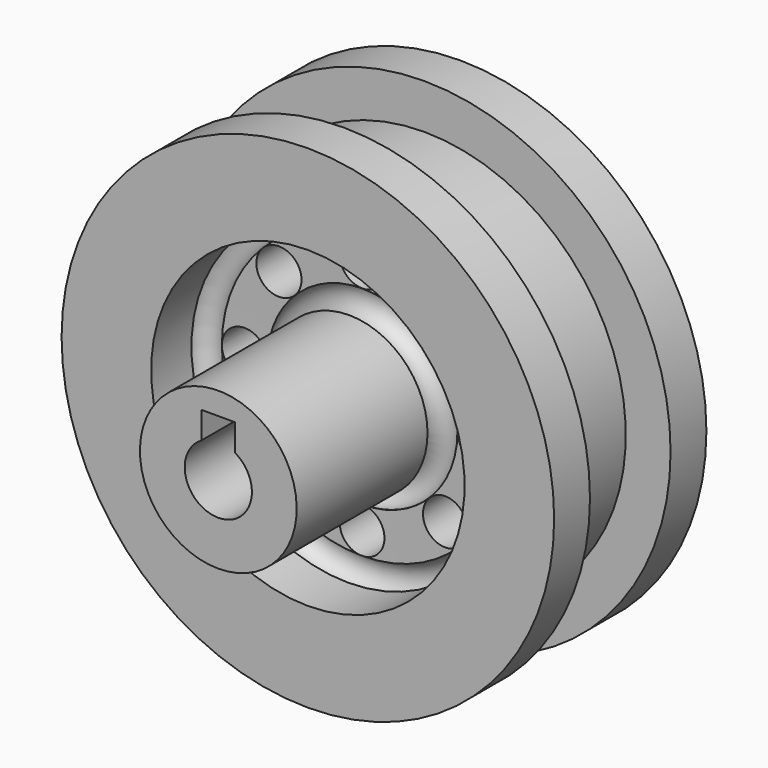
from build123d import *

# Parameters (mm, degrees)
F3_DEPTH        = 27.001
F4_R            = 2
F5_DEPTH        = 20.001
F5_COPIES_COUNT = 8
F6_R            = 1.5
F6_R_2          = 1.495


# Not quite as in the source:
# - a pattern or mirror of a feature is missing from the dataset's text; its kind, count and spacing are read off the source's solid


with BuildPart() as f1:
    # F0 (on Right) → F1 (revolve)
    with BuildSketch(Plane.YZ):
        Polygon((-11.6093918758, -7), (4.4935383189, -7), (4.3906081242, -13.9992432002), (-1.6093918758, -13.9992432002), (-1.6093918758, -21.9992432002), (2.3906081242, -21.9992432002), (2.3906081242, -17.9992432002), (11.3906081242, -17.9992432002), (11.3906081242, -21.9992432002), (15.3906081242, -21.9992432002), (15.3906081242, -13.9992432002), (8.3906081242, -13.9992432002), (8.3906081242, -7), (11.3906081242, -7), (11.3906081242, -3), (-11.6093918758, -3), align=None)
    revolve(axis=Axis((0, -0.5103430335, 0), (0, 1, 0)))

    # F2 (on face) → F3 (cut, through all)
    with BuildSketch(Plane.XZ.offset(11.6093918758)):
        with BuildLine():
            Line((-1.5, 5), (-1.5, 2.5980762114))
            ThreePointArc((-1.5, 2.5980762114), (0, 3), (1.5, 2.5980762114))
            Line((1.5, 2.5980762114), (1.5, 5))
            Line((1.5, 5), (-1.5, 5))
        make_face()
        with BuildLine():
            Line((-1.5, 2.5980762114), (-1.5, 0))
            Line((-1.5, 0), (1.5, 0))
            Line((1.5, 0), (1.5, 2.5980762114))
            ThreePointArc((1.5, 2.5980762114), (0, 3), (-1.5, 2.5980762114))
        make_face()
    extrude(amount=-F3_DEPTH, mode=Mode.SUBTRACT)

    # F4 (on face) → F5 (cut, through all)
    with BuildSketch(Plane(origin=(0, 8.3906081242, 0), x_dir=(-1, 0, 0), z_dir=(0, 1, 0))):
        with Locations((-10.5, 0)):
            Circle(F4_R)
    f5 = extrude(amount=-F5_DEPTH, mode=Mode.SUBTRACT)

    # F5_copies: F5 ×8 about axis
    f5_copies_axis = Axis((0, 0, 0), (0, 1, 0))
    for i in range(1, F5_COPIES_COUNT):
        add(f5.rotate(f5_copies_axis, i * 360 / F5_COPIES_COUNT), mode=Mode.SUBTRACT)

    # F7: sweep along a path in F7_path
    with BuildLine(Plane(origin=(0, 4.3906081242, -13.9992432002), x_dir=(0, 0, 1), z_dir=(0, -1, 0))) as f7_path:
        CenterArc((13.9992432002, 0), 13.9992432002, 0, 360)
    # F6 (on Top) → F7 (sweep, cut)
    with BuildSketch(Plane.XY):
        with Locations((13.9992432002, 4.3906081242)):
            Circle(F6_R)
        with Locations((7, 4.4935383189)):
            Circle(F6_R_2)
    sweep(path=f7_path.line, mode=Mode.SUBTRACT)


solid = f1.part
